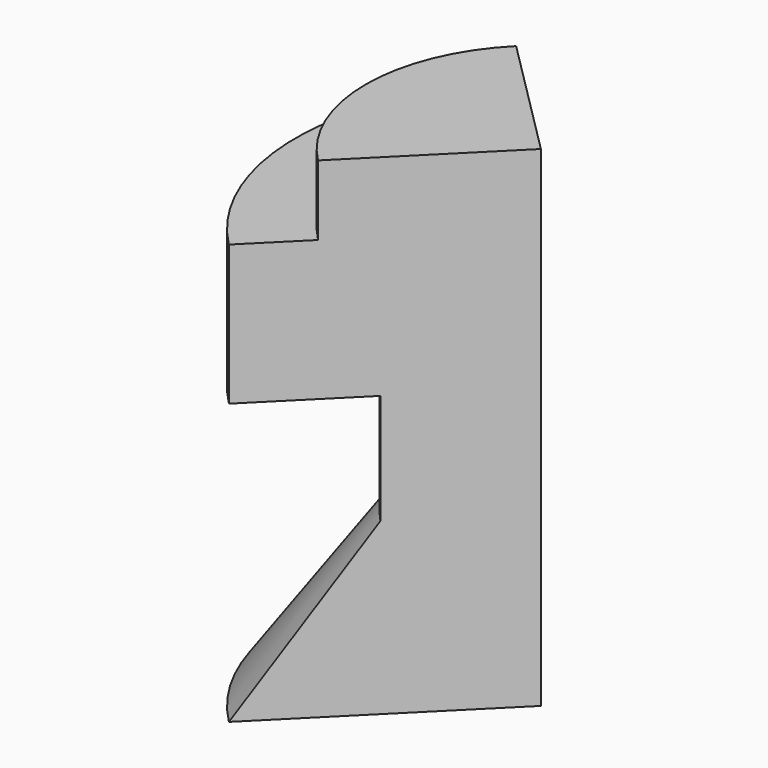
from build123d import *

# Parameters (mm, degrees)
F1_ANGLE_BACK = 45
F1_ANGLE      = 90


# Not quite as in the source:
# - a feature of the source that left no trace in its solid (it failed there, or was rolled back) is left out


with BuildPart() as f1:
    # F0 (on Front) → F1 (revolve)
    with BuildSketch(Plane.XZ, mode=Mode.PRIVATE) as f1_sk:
        Polygon((0, 40), (-25, 40), (-25, 30), (-35, 30), (-35, 10), (-18, 10), (-18, -5.7214838854), (-35, -30), (0, -30), align=None)
    revolve(f1_sk.sketch.rotate(Axis((0, 0, 5), (0, 0, 1)), -F1_ANGLE_BACK), axis=Axis((0, 0, 5), (0, 0, 1)), revolution_arc=F1_ANGLE)


solid = f1.part
